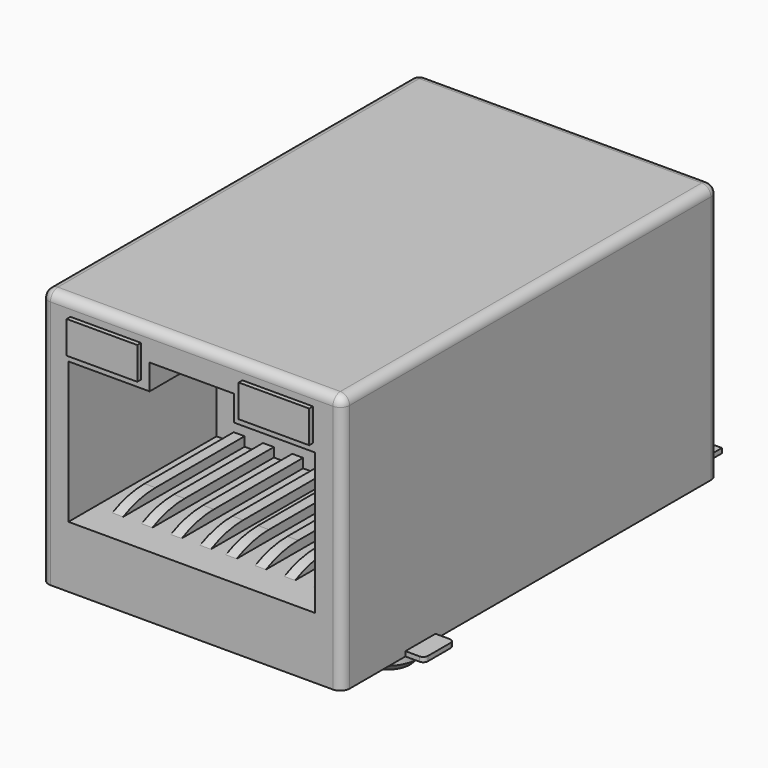
from build123d import *

# Parameters (mm, degrees)
F0_W          = 16.256
F0_H          = 25.4
F1_DEPTH      = 13.97
F2_R          = 0.5
F4_DEPTH      = 10
F5_W          = 0.5874776107
F5_H          = 8.6386585608
F6_DEPTH      = 0.5
F7_T1_DEPTH   = 11.4847249695
F7_2_T1_DEPTH = 11.4847249695
F7_3_T1_DEPTH = 11.4847249695
F7_4_T1_DEPTH = 11.4847249695
F7_5_T1_DEPTH = 11.4847249695
F7_6_T1_DEPTH = 11.4847249695
F7_7_T1_DEPTH = 11.4847249695
F7_8_T1_DEPTH = 11.4847249695
F8_R          = 1.5875
F9_DEPTH      = 0.9906
F10_W         = 0.6096
F10_H         = 1.778
F10_W_2       = 0.762
F11_DEPTH     = 0.254
F12_W         = 3.8125803694
F12_H         = 1.7465446144
F13_DEPTH     = 0.254
F14_SIZE      = 0.381


# Not quite as in the source:
# - a fillet or chamfer that OpenCascade refuses, or shapes differently, is made with other operations: its cross-section is extruded or revolved along the edge and cut away or added


with BuildPart() as f1:
    # F0 (on Top) → F1 (new body)
    with BuildSketch(Plane.XY):
        Rectangle(F0_W, F0_H)
    extrude(amount=F1_DEPTH)

    # F2
    f2_edges = [f1.edges().sort_by_distance(p)[0] for p in [
        (8.128, 12.7, 6.985),
        (-8.128, 12.7, 6.985),
        (0, -12.7, 13.97),
        (-8.128, 0, 13.97),
        (0, 12.7, 13.97),
        (8.128, 0, 13.97),
        (-8.128, -12.7, 6.985),
        (8.128, -12.7, 6.985),
    ]]
    fillet(f2_edges, radius=F2_R)

    # F3 (on face) → F4 (cut)
    with BuildSketch(Plane.XZ.offset(12.7)):
        Polygon((2.2763202433, 12.331135571), (0, 12.331135571), (-2.2763202433, 12.331135571), (-2.2763202433, 10.9573551454), (-6.6607256886, 10.9573551454), (-6.6607256886, 3.3284908859), (0, 3.3284908859), (6.6607256886, 3.3284908859), (6.6607256886, 10.9573551454), (2.2763202433, 10.9573551454), align=None)
    extrude(amount=-F4_DEPTH, mode=Mode.SUBTRACT)

    # F8 (on face) → F9 (join)
    with BuildSketch(Plane(origin=(0, 0, 0), x_dir=(1, 0, 0), z_dir=(0, 0, -1))):
        with Locations((6.35, 7.4168)):
            Circle(F8_R)
        with Locations((-6.35, 7.4168)):
            Circle(F8_R)
    extrude(amount=F9_DEPTH)

    # F10 (on face) → F11 (join)
    with BuildSketch(Plane(origin=(0, 0, 0), x_dir=(1, 0, 0), z_dir=(0, 0, -1))):
        with Locations((0.508, -13.5128)):
            Rectangle(F10_W, F10_H)
        with Locations((1.524, -13.5128)):
            Rectangle(F10_W, F10_H)
        with Locations((2.54, -13.5128)):
            Rectangle(F10_W, F10_H)
        with Locations((3.556, -13.5128)):
            Rectangle(F10_W, F10_H)
        with Locations((4.7498, -13.5128)):
            Rectangle(F10_W_2, F10_H)
        with Locations((6.5786, -13.5128)):
            Rectangle(F10_W_2, F10_H)
        with Locations((-0.508, -13.5128)):
            Rectangle(F10_W, F10_H)
        with Locations((-2.54, -13.5128)):
            Rectangle(F10_W, F10_H)
        with Locations((-1.524, -13.5128)):
            Rectangle(F10_W, F10_H)
        with Locations((-3.556, -13.5128)):
            Rectangle(F10_W, F10_H)
        with Locations((-4.7498, -13.5128)):
            Rectangle(F10_W_2, F10_H)
        with Locations((-6.5786, -13.5128)):
            Rectangle(F10_W_2, F10_H)
        with BuildLine():
            Line((8.89, 8.4328), (8.128, 8.4328))
            Line((8.128, 8.4328), (8.128, 6.4008))
            Line((8.128, 6.4008), (8.89, 6.4008))
            ThreePointArc((8.89, 6.4008), (9.0696051224, 6.4751948776), (9.144, 6.6548))
            Line((9.144, 6.6548), (9.144, 8.1788))
            ThreePointArc((9.144, 8.1788), (9.0696051224, 8.3584051224), (8.89, 8.4328))
        make_face()
        with BuildLine():
            ThreePointArc((-8.89, 8.4328), (-9.0696051224, 8.3584051224), (-9.144, 8.1788))
            Line((-9.144, 8.1788), (-9.144, 6.6548))
            ThreePointArc((-9.144, 6.6548), (-9.0696051224, 6.4751948776), (-8.89, 6.4008))
            Line((-8.89, 6.4008), (-8.128, 6.4008))
            Line((-8.128, 6.4008), (-8.128, 8.4328))
            Line((-8.128, 8.4328), (-8.89, 8.4328))
        make_face()
    extrude(amount=-F11_DEPTH)

    # F14
    f14_edges = [f1.edges().sort_by_distance(p)[0] for p in [
        (4.7625, -7.4168, -0.9906),
        (-7.9375, -7.4168, -0.9906),
    ]]
    chamfer(f14_edges, length=F14_SIZE)


with BuildPart() as f6:
    # F5 (on face) → F6 (new body)
    with BuildSketch(Plane.XY.offset(3.3284908859)):
        with Locations((0.6958528975, -6.5825465135)):
            Rectangle(F5_W, F5_H)
    extrude(amount=F6_DEPTH)

    # F7: fillet of radius 5 on 1 edges, made by hand

    # F7_s2 → F7_t1 (cut)
    with BuildSketch(Plane.YZ.offset(-5.0465095873)):
        with BuildLine():
            ThreePointArc((-10.9018757939, 3.3284908859), (-9.8404603109, 3.7018880583), (-8.7224263222, 3.8284908859))
            Line((-8.7224263222, 3.8284908859), (-10.9018757939, 3.8284908859))
            Line((-10.9018757939, 3.8284908859), (-10.9018757939, 3.3284908859))
        make_face()
    extrude(amount=F7_T1_DEPTH, mode=Mode.SUBTRACT)


with BuildPart() as f6b:
    # F5 (on face) → F6, piece 2 (new body)
    with BuildSketch(Plane.XY.offset(3.3284908859)):
        with Locations((2.2758528975, -6.5825465135)):
            Rectangle(F5_W, F5_H)
    extrude(amount=F6_DEPTH)

    # F7#2: fillet of radius 5 on 1 edges, made by hand

    # F7_2_s2 → F7_2_t1 (cut)
    with BuildSketch(Plane.YZ.offset(-3.4665095873)):
        with BuildLine():
            ThreePointArc((-10.9018757939, 3.3284908859), (-9.8404603109, 3.7018880583), (-8.7224263222, 3.8284908859))
            Line((-8.7224263222, 3.8284908859), (-10.9018757939, 3.8284908859))
            Line((-10.9018757939, 3.8284908859), (-10.9018757939, 3.3284908859))
        make_face()
    extrude(amount=F7_2_T1_DEPTH, mode=Mode.SUBTRACT)


with BuildPart() as f6c:
    # F5 (on face) → F6, piece 3 (new body)
    with BuildSketch(Plane.XY.offset(3.3284908859)):
        with Locations((3.8558528975, -6.5825465135)):
            Rectangle(F5_W, F5_H)
    extrude(amount=F6_DEPTH)

    # F7#3: fillet of radius 5 on 1 edges, made by hand

    # F7_3_s2 → F7_3_t1 (cut)
    with BuildSketch(Plane.YZ.offset(-1.8865095873)):
        with BuildLine():
            ThreePointArc((-10.9018757939, 3.3284908859), (-9.8404603109, 3.7018880583), (-8.7224263222, 3.8284908859))
            Line((-8.7224263222, 3.8284908859), (-10.9018757939, 3.8284908859))
            Line((-10.9018757939, 3.8284908859), (-10.9018757939, 3.3284908859))
        make_face()
    extrude(amount=F7_3_T1_DEPTH, mode=Mode.SUBTRACT)


with BuildPart() as f6d:
    # F5 (on face) → F6, piece 4 (new body)
    with BuildSketch(Plane.XY.offset(3.3284908859)):
        with Locations((5.4358528975, -6.5825465135)):
            Rectangle(F5_W, F5_H)
    extrude(amount=F6_DEPTH)

    # F7#4: fillet of radius 5 on 1 edges, made by hand

    # F7_4_s2 → F7_4_t1 (cut)
    with BuildSketch(Plane.YZ.offset(-0.3065095873)):
        with BuildLine():
            ThreePointArc((-10.9018757939, 3.3284908859), (-9.8404603109, 3.7018880583), (-8.7224263222, 3.8284908859))
            Line((-8.7224263222, 3.8284908859), (-10.9018757939, 3.8284908859))
            Line((-10.9018757939, 3.8284908859), (-10.9018757939, 3.3284908859))
        make_face()
    extrude(amount=F7_4_T1_DEPTH, mode=Mode.SUBTRACT)


with BuildPart() as f6e:
    # F5 (on face) → F6, piece 5 (new body)
    with BuildSketch(Plane.XY.offset(3.3284908859)):
        with Locations((-0.6958528975, -6.5825465135)):
            Rectangle(F5_W, F5_H)
    extrude(amount=F6_DEPTH)

    # F7#5: fillet of radius 5 on 1 edges, made by hand

    # F7_5_s2 → F7_5_t1 (cut)
    with BuildSketch(Plane.YZ.offset(-6.4382153822)):
        with BuildLine():
            ThreePointArc((-10.9018757939, 3.3284908859), (-9.8404603109, 3.7018880583), (-8.7224263222, 3.8284908859))
            Line((-8.7224263222, 3.8284908859), (-10.9018757939, 3.8284908859))
            Line((-10.9018757939, 3.8284908859), (-10.9018757939, 3.3284908859))
        make_face()
    extrude(amount=F7_5_T1_DEPTH, mode=Mode.SUBTRACT)


with BuildPart() as f6f:
    # F5 (on face) → F6, piece 6 (new body)
    with BuildSketch(Plane.XY.offset(3.3284908859)):
        with Locations((-3.8558528975, -6.5825465135)):
            Rectangle(F5_W, F5_H)
    extrude(amount=F6_DEPTH)

    # F7#6: fillet of radius 5 on 1 edges, made by hand

    # F7_6_s2 → F7_6_t1 (cut)
    with BuildSketch(Plane.YZ.offset(-9.5982153822)):
        with BuildLine():
            ThreePointArc((-10.9018757939, 3.3284908859), (-9.8404603109, 3.7018880583), (-8.7224263222, 3.8284908859))
            Line((-8.7224263222, 3.8284908859), (-10.9018757939, 3.8284908859))
            Line((-10.9018757939, 3.8284908859), (-10.9018757939, 3.3284908859))
        make_face()
    extrude(amount=F7_6_T1_DEPTH, mode=Mode.SUBTRACT)


with BuildPart() as f6g:
    # F5 (on face) → F6, piece 7 (new body)
    with BuildSketch(Plane.XY.offset(3.3284908859)):
        with Locations((-2.2758528975, -6.5825465135)):
            Rectangle(F5_W, F5_H)
    extrude(amount=F6_DEPTH)

    # F7#7: fillet of radius 5 on 1 edges, made by hand

    # F7_7_s2 → F7_7_t1 (cut)
    with BuildSketch(Plane.YZ.offset(-8.0182153822)):
        with BuildLine():
            ThreePointArc((-10.9018757939, 3.3284908859), (-9.8404603109, 3.7018880583), (-8.7224263222, 3.8284908859))
            Line((-8.7224263222, 3.8284908859), (-10.9018757939, 3.8284908859))
            Line((-10.9018757939, 3.8284908859), (-10.9018757939, 3.3284908859))
        make_face()
    extrude(amount=F7_7_T1_DEPTH, mode=Mode.SUBTRACT)


with BuildPart() as f6h:
    # F5 (on face) → F6, piece 8 (new body)
    with BuildSketch(Plane.XY.offset(3.3284908859)):
        with Locations((-5.4358528975, -6.5825465135)):
            Rectangle(F5_W, F5_H)
    extrude(amount=F6_DEPTH)

    # F7#8: fillet of radius 5 on 1 edges, made by hand

    # F7_8_s2 → F7_8_t1 (cut)
    with BuildSketch(Plane.YZ.offset(-11.1782153822)):
        with BuildLine():
            ThreePointArc((-10.9018757939, 3.3284908859), (-9.8404603109, 3.7018880583), (-8.7224263222, 3.8284908859))
            Line((-8.7224263222, 3.8284908859), (-10.9018757939, 3.8284908859))
            Line((-10.9018757939, 3.8284908859), (-10.9018757939, 3.3284908859))
        make_face()
    extrude(amount=F7_8_T1_DEPTH, mode=Mode.SUBTRACT)


with BuildPart() as f13:
    # F12 (on face) → F13 (new body)
    with BuildSketch(Plane.XZ.offset(12.7)):
        with Locations((-4.6439180151, 12.2411930934)):
            Rectangle(F12_W, F12_H)
    extrude(amount=F13_DEPTH)


with BuildPart() as f13b:
    # F12 (on face) → F13, piece 2 (new body)
    with BuildSketch(Plane.XZ.offset(12.7)):
        with Locations((4.6439180151, 12.2411930934)):
            Rectangle(F12_W, F12_H)
    extrude(amount=F13_DEPTH)


solid = Compound([f1.part, f6.part, f6b.part, f6c.part, f6d.part, f6e.part, f6f.part, f6g.part, f6h.part, f13.part, f13b.part])
